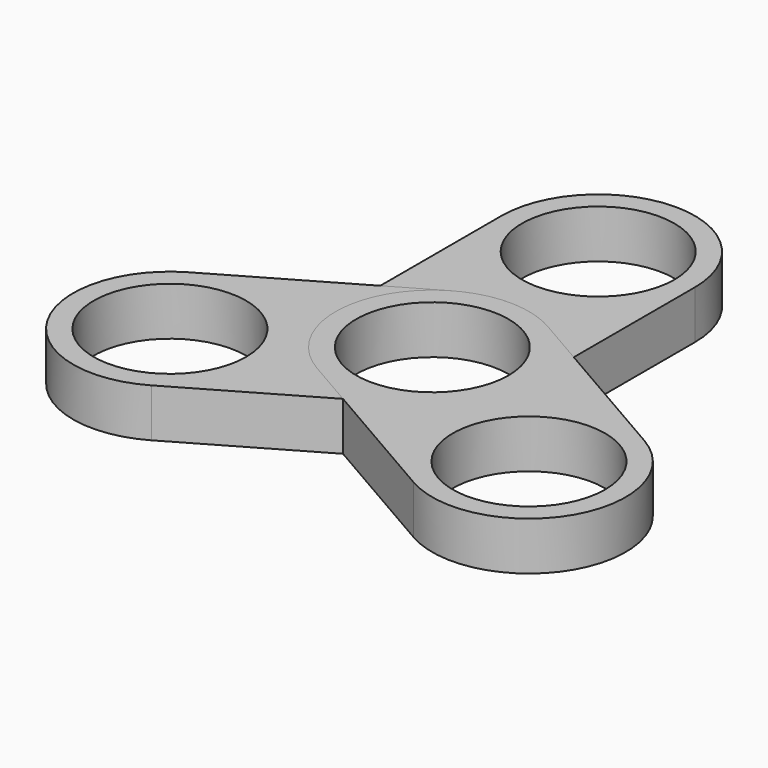
from build123d import *

# Parameters (mm, degrees)
F1_DEPTH        = 7
F1_COPIES_COUNT = 3


# Not quite as in the source:
# - a feature of the source that left no trace in its solid (it failed there, or was rolled back) is left out
# - a pattern or mirror of a feature is missing from the dataset's text; its kind, count and spacing are read off the source's solid


with BuildPart() as f1:
    # F0 (on Top) → F1 (new body)
    with BuildSketch(Plane.XY):
        with BuildLine():
            Line((25.025, 30), (28, 30))
            ThreePointArc((28, 30), (14, 44), (0, 30))
            Line((0, 30), (2.975, 30))
            ThreePointArc((2.975, 30), (14, 41.025), (25.025, 30))
        make_face()
        with BuildLine():
            ThreePointArc((0, 30), (14, 16), (28, 30))
            Line((28, 30), (25.025, 30))
            ThreePointArc((25.025, 30), (14, 18.975), (2.975, 30))
            Line((2.975, 30), (0, 30))
        make_face()
        with BuildLine():
            ThreePointArc((0, 0), (14, 14), (28, 0))
            Line((28, 0), (28, 30))
            ThreePointArc((28, 30), (14, 16), (0, 30))
            Line((0, 30), (0, 0))
        make_face()
        with BuildLine():
            ThreePointArc((2.975, 0), (14, 11.025), (25.025, 0))
            Line((25.025, 0), (28, 0))
            ThreePointArc((28, 0), (14, 14), (0, 0))
            Line((0, 0), (2.975, 0))
        make_face()
        with BuildLine():
            Line((28, 0), (25.025, 0))
            ThreePointArc((25.025, 0), (14, -11.025), (2.975, 0))
            Line((2.975, 0), (0, 0))
            ThreePointArc((0, 0), (14, -14), (28, 0))
        make_face()
    extrude(amount=F1_DEPTH)


with BuildPart() as f1_copies_1:
    # F1_copies: instance of F1
    add(f1.part.rotate(Axis((14, 0, 0), (0, 0, 1)), 1 * 360 / F1_COPIES_COUNT))


with BuildPart() as f1_copies_2:
    # F1_copies: instance of F1
    add(f1.part.rotate(Axis((14, 0, 0), (0, 0, 1)), 2 * 360 / F1_COPIES_COUNT))


solid = Compound([f1.part, f1_copies_1.part, f1_copies_2.part])
